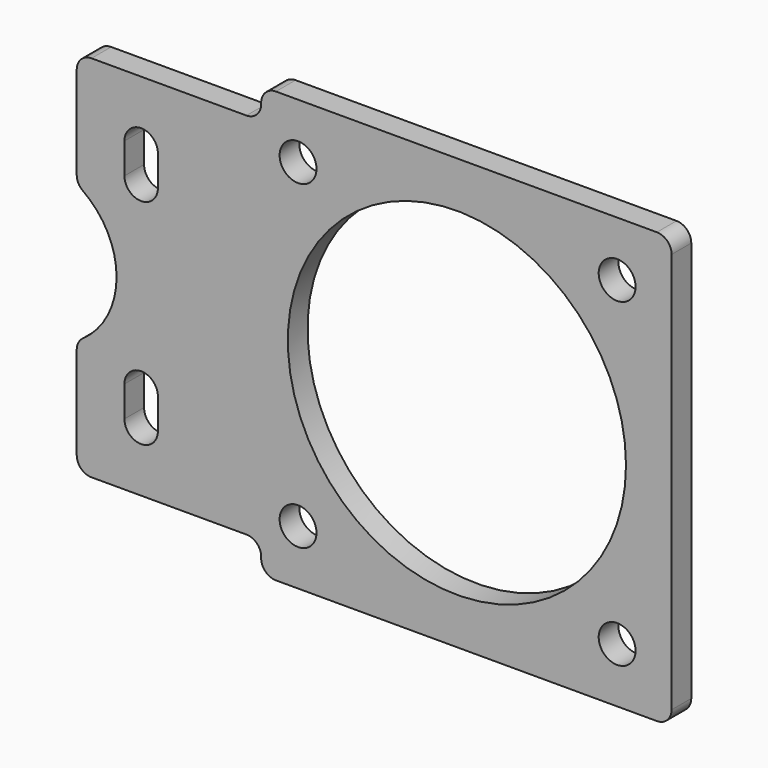
from build123d import *

# Parameters (mm, degrees)
F0_W     = 30.48
F0_H     = 2.54
F1_DEPTH = 44.45
F0_W_2   = 30.9626
F3_DEPTH = 44.45
F4_R     = 1.905
F4_R_2   = 17.4625
F5_DEPTH = 25.4
F2_W     = 19.05
F2_H     = 3.175
F6_DEPTH = 25.4
F7_R     = 1.524


# Not quite as in the source:
# - a feature names something its author has since deleted; it is built from what else it names


with BuildPart() as f1:
    # F0 (on Top) → F1 (new body)
    with BuildSketch(Plane.XY):
        with Locations((-15.24, 1.27)):
            Rectangle(F0_W, F0_H)
    extrude(amount=F1_DEPTH)

    # F0 (on Top) → F3 (join)
    with BuildSketch(Plane.XY):
        with Locations((15.4813, 1.27)):
            Rectangle(F0_W_2, F0_H)
    extrude(amount=F3_DEPTH)

    # F4 (on face) + F2 (on face) → F5 (cut)
    with BuildSketch(Plane.XZ):
        with Locations((-7.62, 38.7731)):
            Circle(F4_R)
        with Locations((-7.62, 5.6769)):
            Circle(F4_R)
        with Locations((25.3365, 38.7731)):
            Circle(F4_R)
        with Locations((25.3365, 5.6769)):
            Circle(F4_R)
        with Locations((8.7884, 22.225)):
            Circle(F4_R_2)
    with BuildSketch(Plane.XZ):
        with BuildLine():
            Line((-22.098, 9.5885), (-22.098, 12.7635))
            ThreePointArc((-22.098, 12.7635), (-23.8252, 14.4907), (-25.5524, 12.7635))
            Line((-25.5524, 12.7635), (-25.5524, 9.5885))
            ThreePointArc((-25.5524, 9.5885), (-23.8252, 7.8613), (-22.098, 9.5885))
        make_face()
        with BuildLine():
            Line((-22.098, 31.6865), (-22.098, 34.8615))
            ThreePointArc((-22.098, 34.8615), (-23.8252, 36.5887), (-25.5524, 34.8615))
            Line((-25.5524, 34.8615), (-25.5524, 31.6865))
            ThreePointArc((-25.5524, 31.6865), (-23.8252, 29.9593), (-22.098, 31.6865))
        make_face()
        with BuildLine():
            Line((-30.48, 29.337), (-30.48, 15.113))
            ThreePointArc((-30.48, 15.113), (-26.3652, 22.225), (-30.48, 29.337))
        make_face()
    extrude(amount=-F5_DEPTH, mode=Mode.SUBTRACT)

    # F2 (on face) → F6 (cut)
    with BuildSketch(Plane.XZ):
        with Locations((-20.955, 42.8625)):
            Rectangle(F2_W, F2_H)
        with Locations((-20.955, 1.5875)):
            Rectangle(F2_W, F2_H)
    extrude(amount=-F6_DEPTH, mode=Mode.SUBTRACT)

    # F7
    f7_edges = [f1.edges().sort_by_distance(p)[0] for p in [
        (-11.43, 1.27, 41.275),
        (-11.43, 1.27, 44.45),
        (-11.43, 1.27, 0),
        (-11.43, 1.27, 3.175),
        (-30.48, 1.27, 3.175),
        (-30.48, 1.27, 29.337),
        (-30.48, 1.27, 15.113),
        (-30.48, 1.27, 41.275),
        (30.9626, 1.27, 0),
        (30.9626, 1.27, 44.45),
    ]]
    fillet(f7_edges, radius=F7_R)


solid = f1.part
